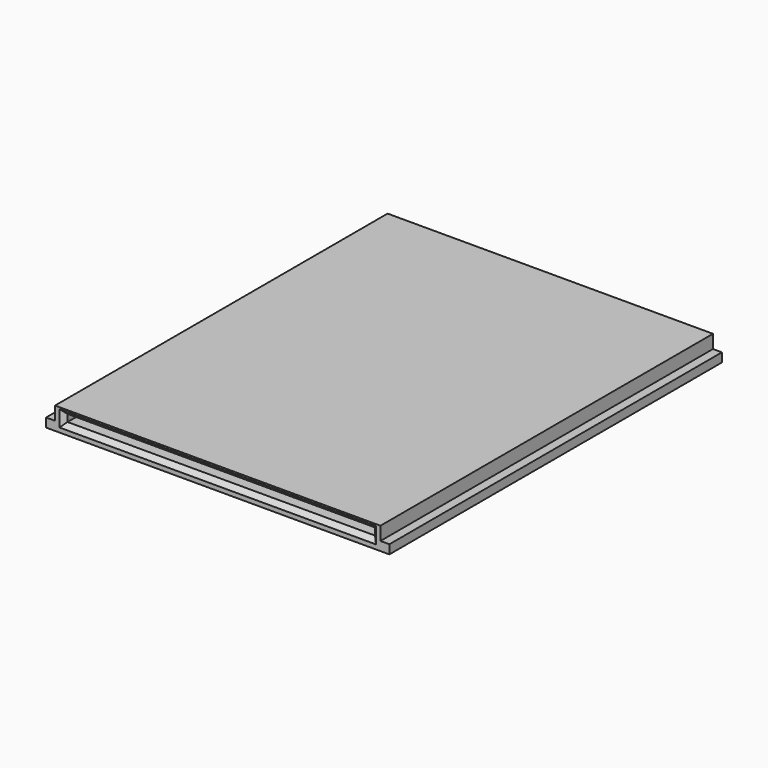
from build123d import *

# Parameters (mm, degrees)
F1_DEPTH = 36.5125
F2_W     = 54.61
F2_H     = 1.27
F3_DEPTH = 1.5875
F4_SIZE  = 0.79374
F5_W     = 25.4
F5_H     = 38.1
F6_DEPTH = 0.254


# Not quite as in the source:
# - a fillet or chamfer is up to 0.001 mm smaller than in the source, because OpenCascade refuses the exact size


with BuildPart() as f1:
    # F0 (on Front) → F1 (new body, symmetric)
    with BuildSketch(Plane.XZ):
        Polygon((27.305, 0), (30.48, 0), (30.48, 1.5875), (28.8925, 1.5875), (28.8925, 3.96875), (0, 3.96875), (0, 2.8575), (27.305, 2.8575), (27.305, 1.5875), (0, 1.5875), (0, 0), align=None)
        Polygon((-27.305, 0), (0, 0), (0, 1.5875), (-27.305, 1.5875), (-27.305, 2.8575), (0, 2.8575), (0, 3.96875), (-28.8925, 3.96875), (-28.8925, 1.5875), (-30.48, 1.5875), (-30.48, 0), align=None)
    extrude(amount=F1_DEPTH, both=True)

    # F2 (on face) → F3 (join)
    with BuildSketch(Plane(origin=(0, 36.5125, 0), x_dir=(-1, 0, 0), z_dir=(0, 1, 0))):
        Polygon((-30.48, 1.5875), (-30.48, 0), (30.48, 0), (30.48, 1.5875), (28.8925, 1.5875), (28.8925, 3.96875), (-28.8925, 3.96875), (-28.8925, 1.5875), align=None)
        with Locations((0, 2.2225)):
            Rectangle(F2_W, F2_H, mode=Mode.SUBTRACT)
        with Locations((0, 2.2225)):
            Rectangle(F2_W, F2_H)
    extrude(amount=F3_DEPTH)

    # F4 (size 0.79375 in the source; OpenCascade refuses exactly that, so slightly less here)
    f4_edges = [f1.edges().sort_by_distance(p)[0] for p in [
        (27.305, -36.5125, 2.2225),
        (0, -36.5125, 1.5875),
        (0, -36.5125, 2.8575),
        (-27.305, -36.5125, 2.2225),
        (29.68625, 38.1, 1.5875),
        (28.8925, 38.1, 2.778125),
        (0, 38.1, 3.96875),
        (0, 38.1, 0),
        (30.48, 38.1, 0.79375),
        (-28.8925, 38.1, 2.778125),
        (-29.68625, 38.1, 1.5875),
        (-30.48, 38.1, 0.79375),
    ]]
    chamfer(f4_edges, length=F4_SIZE)

    # F5 (on face) → F6 (cut)
    with BuildSketch(Plane(origin=(0, 0, 0), x_dir=(1, 0, 0), z_dir=(0, 0, -1))):
        Rectangle(F5_W, F5_H)
    extrude(amount=-F6_DEPTH, mode=Mode.SUBTRACT)


solid = f1.part
